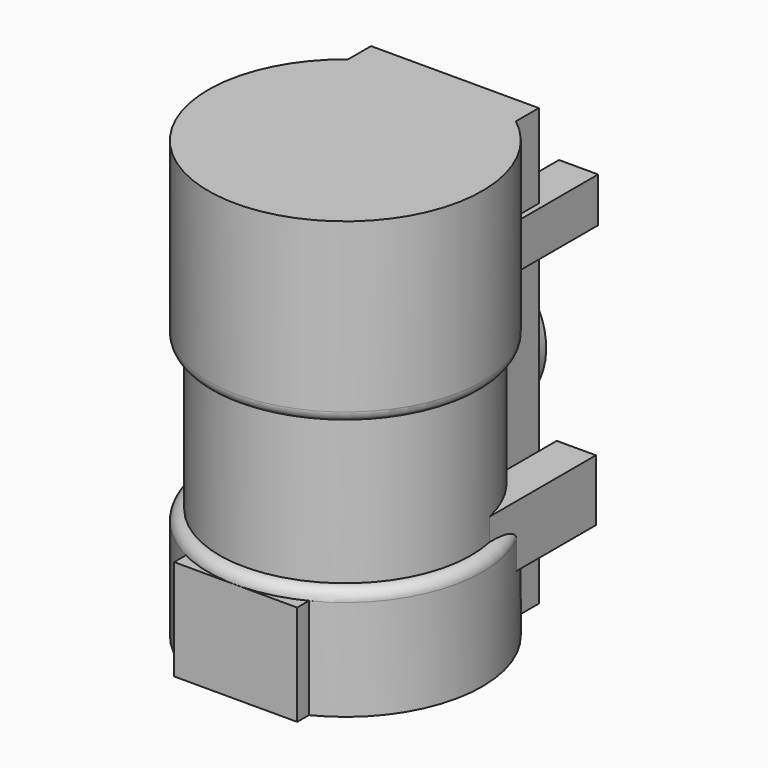
from build123d import *

# Parameters (mm, degrees)
F0_R           = 11.25
F1_DEPTH       = 39
F2_R           = 12.25
F2_R_2         = 11.25
F3_DEPTH       = 16
F5_R           = 0.99999
F4_R           = 12.25
F4_R_2         = 11.25
F6_DEPTH       = 10
F7_R           = 0.99999
F9_DEPTH       = 9
F11_DEPTH      = 39
F12_W          = 3.5
F12_H          = 5.5
F13_DEPTH      = 2
F13_DEPTH_BACK = 12
F15_DEPTH      = 2
F16_W          = 0.5
F16_H          = 4
F16_W_2        = 3
F17_DEPTH      = 6
F17_DEPTH_BACK = 16.7


# Not quite as in the source:
# - a fillet or chamfer is up to 0.001 mm smaller than in the source, because OpenCascade refuses the exact size


with BuildPart() as f1:
    # F0 (on Top) → F1 (new body)
    with BuildSketch(Plane.XY):
        Circle(F0_R)
    extrude(amount=F1_DEPTH)

    # F2 (on face) → F3 (join)
    with BuildSketch(Plane.XY.offset(39)):
        Circle(F2_R)
        Circle(F2_R_2, mode=Mode.SUBTRACT)
    extrude(amount=-F3_DEPTH)

    # F5 (radius 1 in the source; OpenCascade refuses exactly that, so slightly less here)
    f5_edges = [f1.edges().sort_by_distance(p)[0] for p in [
        (-12.25, 0, 23),
    ]]
    fillet(f5_edges, radius=F5_R)

    # F4 (on face) → F6 (join)
    with BuildSketch(Plane(origin=(0, 0, 0), x_dir=(1, 0, 0), z_dir=(0, 0, -1))):
        Circle(F4_R)
        Circle(F4_R_2, mode=Mode.SUBTRACT)
    extrude(amount=-F6_DEPTH)

    # F7 (radius 1 in the source; OpenCascade refuses exactly that, so slightly less here)
    f7_edges = [f1.edges().sort_by_distance(p)[0] for p in [
        (-12.25, 0, 10),
    ]]
    fillet(f7_edges, radius=F7_R)

    # F8 (on face) → F9 (join)
    with BuildSketch(Plane(origin=(0, 0, 0), x_dir=(1, 0, 0), z_dir=(0, 0, -1))):
        with BuildLine():
            Line((0, 12.25), (-5.5, 12.25))
            Line((-5.5, 12.25), (-5.5, 10.9458896395))
            ThreePointArc((-5.5, 10.9458896395), (-2.8262476817, 11.9195144214), (0, 12.25))
        make_face()
        with BuildLine():
            Line((5.5, 12.25), (0, 12.25))
            ThreePointArc((0, 12.25), (2.8262476817, 11.9195144214), (5.5, 10.9458896395))
            Line((5.5, 10.9458896395), (5.5, 12.25))
        make_face()
    extrude(amount=-F9_DEPTH)

    # F10 (on face) → F11 (join)
    with BuildSketch(Plane(origin=(0, 0, 0), x_dir=(1, 0, 0), z_dir=(0, 0, -1))):
        with BuildLine():
            Line((7.5, -12.25), (7.5, -9.6856853139))
            ThreePointArc((7.5, -9.6856853139), (3.9631335396, -11.5912066907), (0, -12.25))
            Line((0, -12.25), (7.5, -12.25))
        make_face()
        with BuildLine():
            ThreePointArc((0, -12.25), (-3.9631335396, -11.5912066907), (-7.5, -9.6856853139))
            Line((-7.5, -9.6856853139), (-7.5, -12.25))
            Line((-7.5, -12.25), (0, -12.25))
        make_face()
        with BuildLine():
            Line((7.5, -8.25), (-7.5, -8.25))
            Line((-7.5, -8.25), (-7.5, -9.6856853139))
            ThreePointArc((-7.5, -9.6856853139), (-3.9631335396, -11.5912066907), (0, -12.25))
            ThreePointArc((0, -12.25), (3.9631335396, -11.5912066907), (7.5, -9.6856853139))
            Line((7.5, -9.6856853139), (7.5, -8.25))
        make_face()
    extrude(amount=-F11_DEPTH)

    # F12 (on face) → F13 (join, two sides)
    with BuildSketch(Plane(origin=(0, 12.25, 0), x_dir=(-1, 0, 0), z_dir=(0, 1, 0))) as f13_sk:
        with Locations((-9.25, 9.25)):
            Rectangle(F12_W, F12_H)
    extrude(amount=F13_DEPTH)
    extrude(f13_sk.sketch, amount=-F13_DEPTH_BACK)

    # F14 (on face) → F15 (join)
    with BuildSketch(Plane(origin=(0, 12.25, 0), x_dir=(-1, 0, 0), z_dir=(0, 1, 0))):
        with BuildLine():
            ThreePointArc((0, 25.4997491551), (-4.6734438866, 14.4240399421), (6.4428955234, 19))
            ThreePointArc((6.4428955234, 19), (4.5592349335, 23.5759600579), (0, 25.4997491551))
        make_face()
    extrude(amount=F15_DEPTH)

    # F16 (on face) → F17 (join, two sides)
    with BuildSketch(Plane(origin=(0, 12.25, 0), x_dir=(-1, 0, 0), z_dir=(0, 1, 0))) as f17_sk:
        with Locations((-7.75, 29.5)):
            Rectangle(F16_W, F16_H)
        with Locations((-6, 29.5)):
            Rectangle(F16_W_2, F16_H)
    extrude(amount=F17_DEPTH)
    extrude(f17_sk.sketch, amount=-F17_DEPTH_BACK)


solid = f1.part
